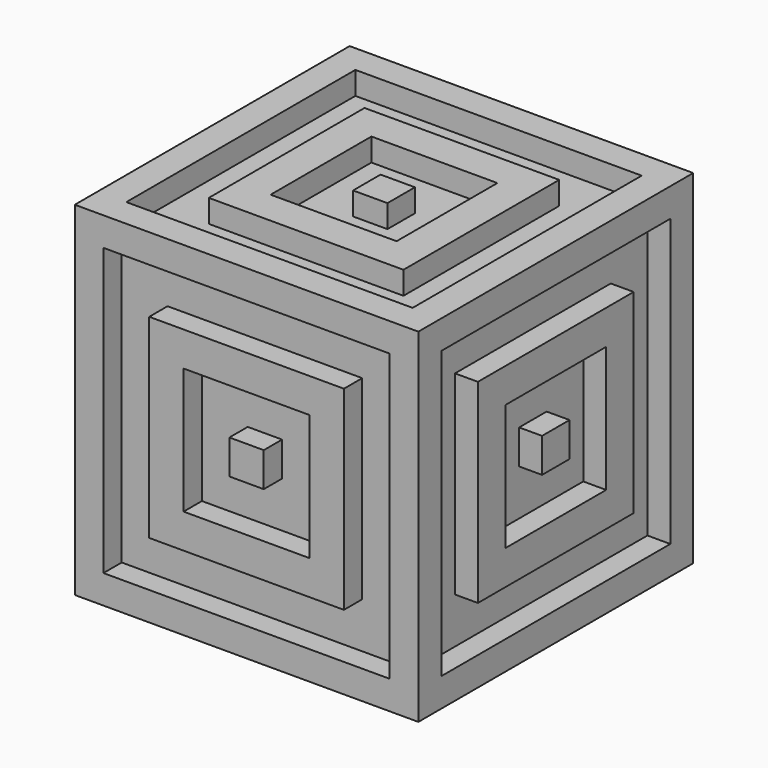
from build123d import *

# Parameters (mm, degrees)
F0_W      = 30
F0_H      = 30
F1_DEPTH  = 30
F2_W      = 25
F2_H      = 25
F2_W_2    = 17
F2_H_2    = 17
F2_W_3    = 11
F2_H_3    = 11
F2_W_4    = 3
F2_H_4    = 3
F3_DEPTH  = 2
F4_W      = 25
F4_H      = 25
F4_W_2    = 17
F4_H_2    = 17
F4_W_3    = 11
F4_H_3    = 11
F4_W_4    = 3
F4_H_4    = 3
F5_DEPTH  = 2
F6_W      = 25
F6_H      = 25
F6_W_2    = 17
F6_H_2    = 17
F6_W_3    = 11
F6_H_3    = 11
F6_W_4    = 3
F6_H_4    = 3
F7_DEPTH  = 2
F8_W      = 25
F8_H      = 25
F8_W_2    = 17
F8_H_2    = 17
F8_W_3    = 11
F8_H_3    = 11
F8_W_4    = 3
F8_H_4    = 3
F9_DEPTH  = 2
F10_W     = 25
F10_H     = 25
F10_W_2   = 17
F10_H_2   = 17
F10_W_3   = 11
F10_H_3   = 11
F10_W_4   = 3
F10_H_4   = 3
F11_DEPTH = 2
F12_W     = 25
F12_H     = 25
F12_W_2   = 17
F12_H_2   = 17
F12_W_3   = 11
F12_H_3   = 11
F12_W_4   = 3
F12_H_4   = 3
F13_DEPTH = 2


# Not quite as in the source:
# - a feature names something its author has since deleted; it is built from what else it names


with BuildPart() as f1:
    # F0 (on Front) → F1 (new body)
    with BuildSketch(Plane.XZ):
        Rectangle(F0_W, F0_H)
    extrude(amount=F1_DEPTH)

    # F2 (on face) → F3 (cut)
    with BuildSketch(Plane.XY.offset(15)):
        with Locations((0, -15)):
            Rectangle(F2_W, F2_H)
        with Locations((0, -15)):
            Rectangle(F2_W_2, F2_H_2, mode=Mode.SUBTRACT)
        with Locations((0, -15)):
            Rectangle(F2_W_3, F2_H_3)
        with Locations((0, -15)):
            Rectangle(F2_W_4, F2_H_4, mode=Mode.SUBTRACT)
    extrude(amount=-F3_DEPTH, mode=Mode.SUBTRACT)

    # F4 (on face) → F5 (cut)
    with BuildSketch(Plane(origin=(-15, 0, 0), x_dir=(0, -1, 0), z_dir=(-1, 0, 0))):
        with Locations((15, 0)):
            Rectangle(F4_W, F4_H)
        with Locations((15, 0)):
            Rectangle(F4_W_2, F4_H_2, mode=Mode.SUBTRACT)
        with Locations((15, 0)):
            Rectangle(F4_W_3, F4_H_3)
        with Locations((15, 0)):
            Rectangle(F4_W_4, F4_H_4, mode=Mode.SUBTRACT)
    extrude(amount=-F5_DEPTH, mode=Mode.SUBTRACT)

    # F6 (on face) → F7 (cut)
    with BuildSketch(Plane(origin=(0, 0, -15), x_dir=(1, 0, 0), z_dir=(0, 0, -1))):
        with Locations((0, 15)):
            Rectangle(F6_W, F6_H)
        with Locations((0, 15)):
            Rectangle(F6_W_2, F6_H_2, mode=Mode.SUBTRACT)
        with Locations((0, 15)):
            Rectangle(F6_W_3, F6_H_3)
        with Locations((0, 15)):
            Rectangle(F6_W_4, F6_H_4, mode=Mode.SUBTRACT)
    extrude(amount=-F7_DEPTH, mode=Mode.SUBTRACT)

    # F8 (on face) → F9 (cut)
    with BuildSketch(Plane.XZ.offset(30)):
        Rectangle(F8_W, F8_H)
        Rectangle(F8_W_2, F8_H_2, mode=Mode.SUBTRACT)
        Rectangle(F8_W_3, F8_H_3)
        Rectangle(F8_W_4, F8_H_4, mode=Mode.SUBTRACT)
    extrude(amount=-F9_DEPTH, mode=Mode.SUBTRACT)

    # F10 (on face) → F11 (cut)
    with BuildSketch(Plane(origin=(0, 0, 0), x_dir=(-1, 0, 0), z_dir=(0, 1, 0))):
        Rectangle(F10_W, F10_H)
        Rectangle(F10_W_2, F10_H_2, mode=Mode.SUBTRACT)
        Rectangle(F10_W_3, F10_H_3)
        Rectangle(F10_W_4, F10_H_4, mode=Mode.SUBTRACT)
    extrude(amount=-F11_DEPTH, mode=Mode.SUBTRACT)

    # F12 (on face) → F13 (cut)
    with BuildSketch(Plane.YZ.offset(15)):
        with Locations((-15, 0)):
            Rectangle(F12_W, F12_H)
        with Locations((-15, 0)):
            Rectangle(F12_W_2, F12_H_2, mode=Mode.SUBTRACT)
        with Locations((-15, 0)):
            Rectangle(F12_W_3, F12_H_3)
        with Locations((-15, 0)):
            Rectangle(F12_W_4, F12_H_4, mode=Mode.SUBTRACT)
    extrude(amount=-F13_DEPTH, mode=Mode.SUBTRACT)


solid = f1.part
